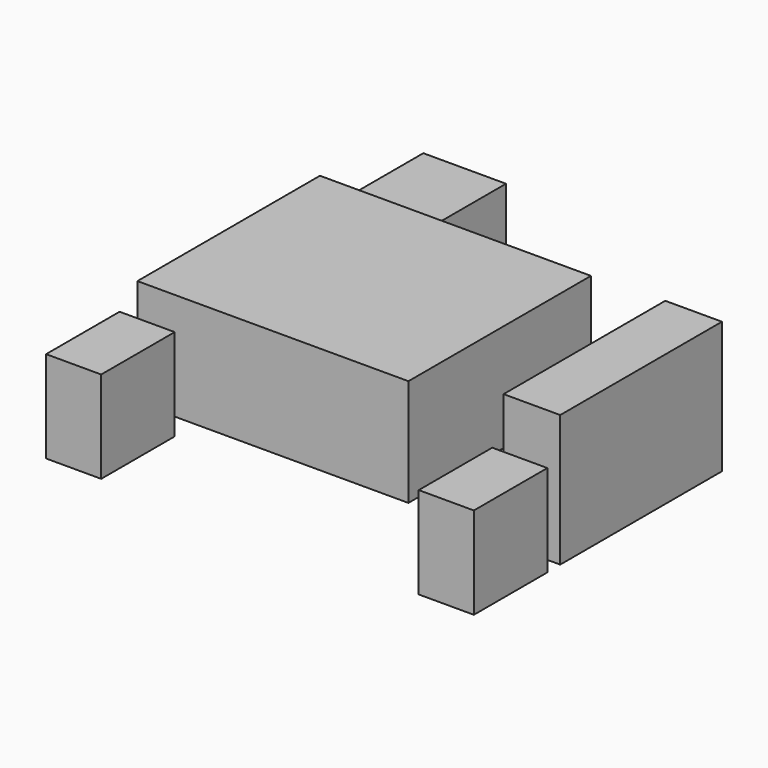
from build123d import *

# Parameters (mm, degrees)
F0_W     = 457.2
F0_H     = 762
F2_DEPTH = 762
F0_W_2   = 2247.9
F0_H_2   = 1892.3
F3_DEPTH = 889
F0_W_3   = 469.9
F0_H_3   = 1676.4
F5_DEPTH = 1092.2
F0_W_4   = 685.8
F0_H_4   = 800.1
F6_DEPTH = 698.5


# Not quite as in the source:
# - the program builds the solid bodies; features that only make, move or delete a surface that nothing else refers to are left out


with BuildPart() as f2:
    # F0 (on Top) → F2 (new body)
    with BuildSketch(Plane.XY):
        with Locations((-1523.4456062317, -1544.3762540817)):
            Rectangle(F0_W, F0_H)
    extrude(amount=F2_DEPTH)


with BuildPart() as f2b:
    # F0 (on Top) → F2, piece 2 (new body)
    with BuildSketch(Plane.XY):
        with Locations((1552.4368286133, -1525.6679058075)):
            Rectangle(F0_W, F0_H)
    extrude(amount=F2_DEPTH)


with BuildPart() as f3:
    # F0 (on Top) → F3 (new body)
    with BuildSketch(Plane.XY):
        with Locations((-654.05, 0)):
            Rectangle(F0_W_2, F0_H_2)
    extrude(amount=F3_DEPTH)


with BuildPart() as f5:
    # F0 (on Top) → F5 (new body)
    with BuildSketch(Plane.XY):
        with Locations((1543.05, -169.3084090948)):
            Rectangle(F0_W_3, F0_H_3)
    extrude(amount=F5_DEPTH)


with BuildPart() as f6:
    # F0 (on Top) → F6 (new body)
    with BuildSketch(Plane.XY):
        with Locations((-1338.3623361588, 1497.0246553421)):
            Rectangle(F0_W_4, F0_H_4)
    extrude(amount=F6_DEPTH)


solid = Compound([f2.part, f2b.part, f3.part, f5.part, f6.part])
